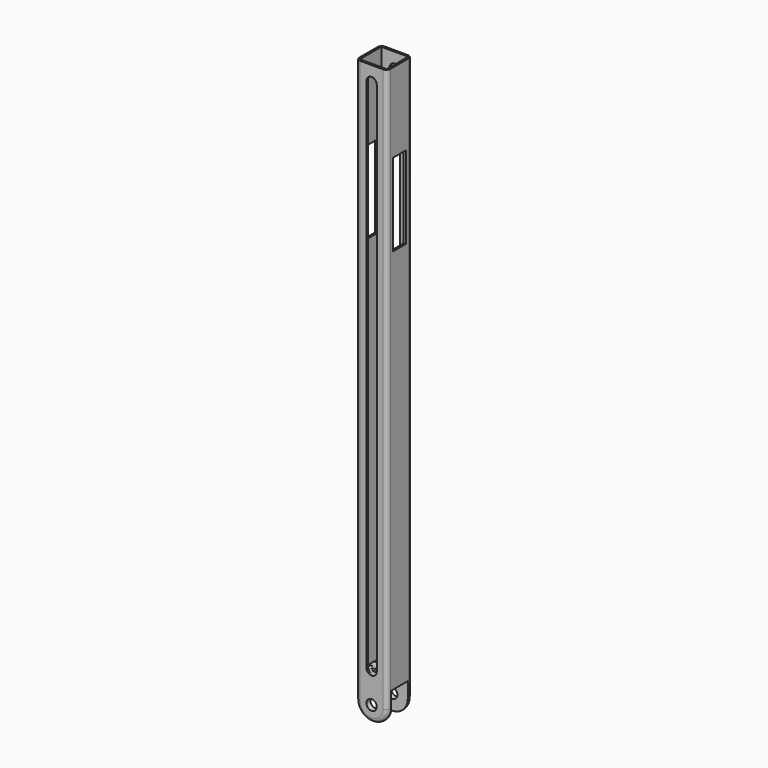
from build123d import *

# Parameters (mm, degrees)
F0_W          = 38.1
F0_H          = 38.1
F1_DEPTH      = 711.2
F2_W          = 16.51
F2_H          = 16.51
F3_DEPTH      = 660.4
F5_DEPTH      = 102.108
F6_W          = 25.4
F6_H          = 38.1
F7_DEPTH      = 55.118
F8_R          = 19.04999
F9_R          = 6.35
F10_DEPTH     = 54.356
F11_W         = 19.3887297064
F11_H         = 101.2880802155
F12_DEPTH     = 118.364
F13_R         = 5.08
F14_TEXT_SIZE = 12.0202491326
F15_DEPTH     = 0.254


# Not quite as in the source:
# - a fillet or chamfer is up to 0.001 mm smaller than in the source, because OpenCascade refuses the exact size
# - Text() gives the source's letters only with a copy of the font that has no kerning and outlines rounded to 1/6400 em; it was checked with that copy


with BuildPart() as f1:
    # F0 (on Top) → F1 (new body)
    with BuildSketch(Plane.XY):
        Rectangle(F0_W, F0_H)
    extrude(amount=F1_DEPTH)

    # F2 (on face) → F3 (cut)
    with BuildSketch(Plane.XY.offset(711.2)):
        with Locations((-8.255, 8.255)):
            Rectangle(F2_W, F2_H)
        with Locations((8.255, 8.255)):
            Rectangle(F2_W, F2_H)
        with Locations((8.255, -8.255)):
            Rectangle(F2_W, F2_H)
        with Locations((-8.255, -8.255)):
            Rectangle(F2_W, F2_H)
    extrude(amount=-F3_DEPTH, mode=Mode.SUBTRACT)

    # F4 (on face) → F5 (cut)
    with BuildSketch(Plane.XZ.offset(19.05)):
        with BuildLine():
            Line((0, 63.5), (0, 685.8))
            ThreePointArc((0, 685.8), (-4.4901280605, 687.6598719395), (-6.35, 692.15))
            Line((-6.35, 692.15), (-6.35, 57.15))
            ThreePointArc((-6.35, 57.15), (-4.4901280605, 61.6401280605), (0, 63.5))
        make_face()
        with BuildLine():
            ThreePointArc((6.35, 692.15), (4.4901280605, 687.6598719395), (0, 685.8))
            Line((0, 685.8), (0, 63.5))
            ThreePointArc((0, 63.5), (4.4901280605, 61.6401280605), (6.35, 57.15))
            Line((6.35, 57.15), (6.35, 692.15))
        make_face()
        with BuildLine():
            ThreePointArc((6.35, 692.15), (4.4901280605, 696.6401280605), (0, 698.5))
            Line((0, 698.5), (0, 685.8))
            ThreePointArc((0, 685.8), (4.4901280605, 687.6598719395), (6.35, 692.15))
        make_face()
        with BuildLine():
            Line((0, 685.8), (0, 698.5))
            ThreePointArc((0, 698.5), (-4.4901280605, 696.6401280605), (-6.35, 692.15))
            ThreePointArc((-6.35, 692.15), (-4.4901280605, 687.6598719395), (0, 685.8))
        make_face()
        with BuildLine():
            Line((0, 50.8), (0, 63.5))
            ThreePointArc((0, 63.5), (-4.4901280605, 61.6401280605), (-6.35, 57.15))
            ThreePointArc((-6.35, 57.15), (-4.4901280605, 52.6598719395), (0, 50.8))
        make_face()
        with BuildLine():
            ThreePointArc((6.35, 57.15), (4.4901280605, 61.6401280605), (0, 63.5))
            Line((0, 63.5), (0, 50.8))
            ThreePointArc((0, 50.8), (4.4901280605, 52.6598719395), (6.35, 57.15))
        make_face()
    extrude(amount=-F5_DEPTH, mode=Mode.SUBTRACT)

    # F6 (on face) → F7 (cut)
    with BuildSketch(Plane.YZ.offset(19.05)):
        with Locations((0, 19.05)):
            Rectangle(F6_W, F6_H)
    extrude(amount=-F7_DEPTH, mode=Mode.SUBTRACT)

    # F8 (radius 19.05 in the source; OpenCascade refuses exactly that, so slightly less here)
    f8_edges = [f1.edges().sort_by_distance(p)[0] for p in [
        (19.05, -15.875, 0),
        (19.05, 15.875, 0),
        (-19.05, -15.875, 0),
        (-19.05, 15.875, 0),
    ]]
    fillet(f8_edges, radius=F8_R)

    # F9 (on face) → F10 (cut)
    with BuildSketch(Plane.XZ.offset(19.05)):
        with Locations((0, 19.05)):
            Circle(F9_R)
    extrude(amount=-F10_DEPTH, mode=Mode.SUBTRACT)

    # F11 (on face) → F12 (cut)
    with BuildSketch(Plane.YZ.offset(19.05)):
        with Locations((0, 562.8330111504)):
            Rectangle(F11_W, F11_H)
    extrude(amount=-F12_DEPTH, mode=Mode.SUBTRACT)

    # F13
    f13_edges = [f1.edges().sort_by_distance(p)[0] for p in [
        (19.05, -19.05, 365.124995),
        (19.05, 19.05, 365.124995),
    ]]
    fillet(f13_edges, radius=F13_R)

    # F14 (on face) → F15 (join)
    with BuildSketch(Plane.XY.offset(50.8)):
        with Locations((-16.51, 5.4437882916)):
            Text('SAH', F14_TEXT_SIZE, font='Open Sans', text_align=(TextAlign.LEFT, TextAlign.BOTTOM))
        with Locations((-16.51, -10.9037505287)):
            Text('DUDE', F14_TEXT_SIZE, font='Open Sans', text_align=(TextAlign.LEFT, TextAlign.BOTTOM))
    extrude(amount=F15_DEPTH)


solid = f1.part
